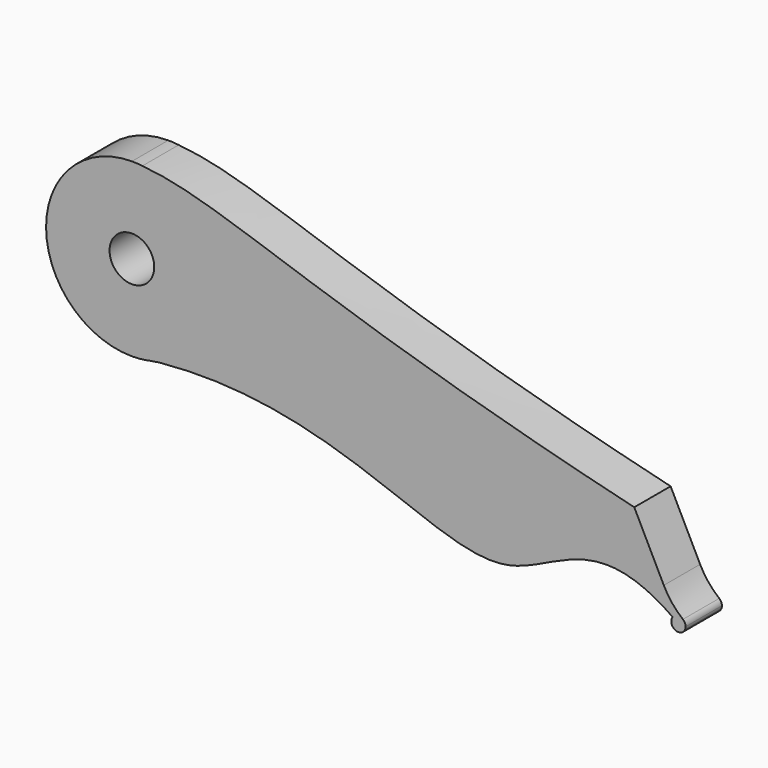
from build123d import *

# Parameters (mm, degrees)
F0_R     = 1.5625
F1_DEPTH = 3.175
F2_R     = 5


# Not quite as in the source:
# - two fillets or chamfers of one size are made in one step
# - a length typed as a fraction of an inch, garbled in the dataset ("3 / 203.2 mm" for 3/8 in), is restored


with BuildPart() as f1:
    # F0 (on Front) → F1 (new body)
    with BuildSketch(Plane.XZ):
        with BuildLine():
            add(Edge.make_bspline(
                [(0, 6), (0.244167608, 5.9909795741), (0.4874256523, 5.9760413709), (0.7309494159, 5.9553096436)],
                knots=[0, 0, 0, 0, 1.4561246163, 1.4561246163, 1.4561246163, 1.4561246163], degree=3))
            ThreePointArc((0, 6), (-6, 0), (0, -6))
            add(Edge.make_bspline(
                [(0, -6), (0.5264900217, -5.918222626), (1.0434262259, -5.850580103), (1.5510661896, -5.7960498338)],
                knots=[0, 0, 0, 0, 0.0231840948, 0.0231840948, 0.0231840948, 0.0231840948], degree=3))
            ThreePointArc((1.5510661896, -5.7960498338), (4.7595376423, -3.6533274465), (6, 0))
            ThreePointArc((6, 0), (4.4936453184, 3.9758208904), (0.7309494159, 5.9553096436))
        make_face()
        Circle(F0_R, mode=Mode.SUBTRACT)
        with BuildLine():
            ThreePointArc((0.7309494159, 5.9553096436), (0.3661571645, 5.9888169893), (0, 6))
            add(Edge.make_bspline(
                [(0, 6), (0.244167608, 5.9909795741), (0.4874256523, 5.9760413709), (0.7309494159, 5.9553096436)],
                knots=[0, 0, 0, 0, 1.4561246163, 1.4561246163, 1.4561246163, 1.4561246163], degree=3))
        make_face()
        with BuildLine():
            add(Edge.make_bspline(
                [(0, -6), (0.5264900217, -5.918222626), (1.0434262259, -5.850580103), (1.5510661896, -5.7960498338)],
                knots=[0, 0, 0, 0, 0.0231840948, 0.0231840948, 0.0231840948, 0.0231840948], degree=3))
            ThreePointArc((0, -6), (0.7822087309, -5.9487939535), (1.5510661896, -5.7960498338))
        make_face()
        with BuildLine():
            add(Edge.make_bspline(
                [(0.7309494159, 5.9553096436), (6.5885872075, 5.4566357259), (12.5999644874, 1.6059529825), (35.1214148104, -3.8675169926)],
                knots=[1.4561246163, 1.4561246163, 1.4561246163, 1.4561246163, 36.4812509364, 36.4812509364, 36.4812509364, 36.4812509364], degree=3))
            ThreePointArc((0.7309494159, 5.9553096436), (4.4936453184, 3.9758208904), (6, 0))
            ThreePointArc((6, 0), (4.7595376423, -3.6533274465), (1.5510661896, -5.7960498338))
            add(Edge.make_bspline(
                [(1.5510661896, -5.7960498338), (14.0781923654, -4.4503961965), (25.6888672866, -15.6775062325), (32.1799724767, -5.7946943127), (37.8041636238, -9.7550129686)],
                knots=[0.0231840948, 0.0231840948, 0.0231840948, 0.0231840948, 0.5953023308, 0.9906507432, 0.9906507432, 0.9906507432, 0.9906507432], degree=3))
            ThreePointArc((37.8041636238, -9.7550129686), (37.8853336655, -9.6677699854), (37.984842679, -9.6022118429))
            Line((37.984842679, -9.6022118429), (35.1214148104, -3.8675169926))
        make_face()
        with BuildLine():
            ThreePointArc((37.984842679, -9.6022118429), (37.8853336655, -9.6677699854), (37.8041636238, -9.7550129686))
            add(Edge.make_bspline(
                [(37.8041636238, -9.7550129686), (37.9371653146, -9.8486671606), (38.0718288537, -9.9467945932), (38.2082048467, -10.0495476698)],
                knots=[0.9906507432, 0.9906507432, 0.9906507432, 0.9906507432, 1, 1, 1, 1], degree=3))
            Line((38.2082048467, -10.0495476698), (37.984842679, -9.6022118429))
        make_face()
        with BuildLine():
            add(Edge.make_bspline(
                [(37.8041636238, -9.7550129686), (37.9371653146, -9.8486671606), (38.0718288537, -9.9467945932), (38.2082048467, -10.0495476698)],
                knots=[0.9906507432, 0.9906507432, 0.9906507432, 0.9906507432, 1, 1, 1, 1], degree=3))
            ThreePointArc((37.8041636238, -9.7550129686), (38.053318778, -10.5249530818), (38.7082048467, -10.0495476698))
            ThreePointArc((38.7082048467, -10.0495476698), (38.4711867055, -9.6242941667), (37.984842679, -9.6022118429))
            Line((37.984842679, -9.6022118429), (38.2082048467, -10.0495476698))
        make_face()
    extrude(amount=F1_DEPTH)

    # F2
    f2_edges = [f1.edges().sort_by_distance(p)[0] for p in [
        (1.551066, -1.5875, -5.79605),
        (37.984843, -1.5875, -9.602212),
    ]]
    fillet(f2_edges, radius=F2_R)


solid = f1.part
